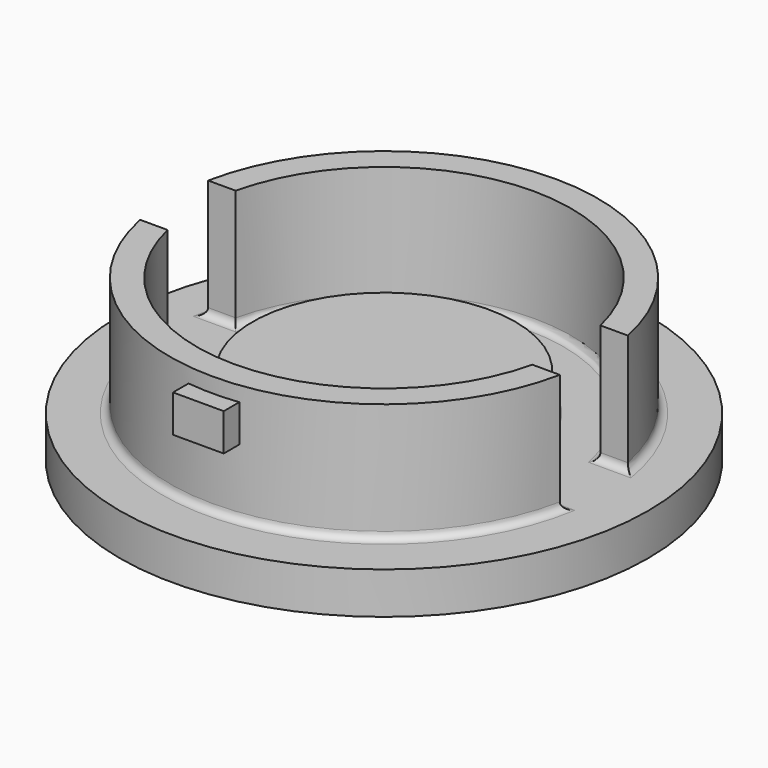
from build123d import *

# Parameters (mm, degrees)
F0_R         = 8.85
F1_DEPTH     = 1.4
F2_R         = 7.175
F2_R_2       = 6.275
F3_DEPTH     = 4
F5_W         = 2.85
F5_H         = 4
F6_DEPTH     = 25
F7_R         = 4.4
F8_DEPTH     = 1.27
F10_W        = 1.7
F10_H        = 1.25
F11_DEPTH    = 0.6
F12_W        = 12.45
F12_H        = 1.85
F13_DEPTH    = 0.8
F14_T1_DEPTH = 6.7489794856
F15_R        = 0.25


# Not quite as in the source:
# - a fillet or chamfer that OpenCascade refuses, or shapes differently, is made with other operations: its cross-section is extruded or revolved along the edge and cut away or added
# - a pattern or mirror of a feature is missing from the dataset's text; its kind, count and spacing are read off the source's solid


with BuildPart() as f1:
    # F0 (on Top) → F1 (new body)
    with BuildSketch(Plane.XY):
        Circle(F0_R)
    extrude(amount=F1_DEPTH)

    # F2 (on face) → F3 (join)
    with BuildSketch(Plane.XY.offset(1.4)):
        Circle(F2_R)
        Circle(F2_R_2, mode=Mode.SUBTRACT)
    extrude(amount=F3_DEPTH)

    # F5 (on offset) → F6 (cut)
    with BuildSketch(Plane.YZ.offset(7.175)):
        with Locations((0, 3.4)):
            Rectangle(F5_W, F5_H)
    extrude(amount=-F6_DEPTH, mode=Mode.SUBTRACT)

    # F7 (on face) → F8 (join)
    with BuildSketch(Plane.XY.offset(1.4)):
        Circle(F7_R)
    extrude(amount=F8_DEPTH)

    # F10 (on offset) → F11 (join, symmetric)
    with BuildSketch(Plane.XZ.offset(7.175)):
        with Locations((0, 4.275)):
            Rectangle(F10_W, F10_H)
    f11 = extrude(amount=F11_DEPTH, both=True)

    # F11_copies: F11 across plane
    add(f11.mirror(Plane.ZX))

    # F12 (on face) → F13 (cut)
    with BuildSketch(Plane(origin=(0, 0, 0), x_dir=(1, 0, 0), z_dir=(0, 0, -1))):
        Rectangle(F12_W, F12_H)
    extrude(amount=-F13_DEPTH, mode=Mode.SUBTRACT)

    # F14: fillet of radius 1 on 2 edges, made by hand

    # F14_s2 → F14_t1 (join)
    with BuildSketch(Plane.XZ.offset(-3.3744897428)):
        with BuildLine():
            ThreePointArc((-6.225, 0), (-5.8776596349, 0.5745966692), (-5.2452041029, 0.8))
            Line((-5.2452041029, 0.8), (-6.225, 0.8))
            Line((-6.225, 0.8), (-6.225, 0))
        make_face()
        with BuildLine():
            ThreePointArc((6.225, 0), (5.8776596349, 0.5745966692), (5.2452041029, 0.8))
            Line((5.2452041029, 0.8), (6.225, 0.8))
            Line((6.225, 0.8), (6.225, 0))
        make_face()
    extrude(amount=F14_T1_DEPTH)

    # F15
    f15_edges = [f1.edges().sort_by_distance(p)[0] for p in [
        (0, 6.275, 1.4),
        (6.571562, 1.425, 1.4),
        (-6.571562, 1.425, 1.4),
        (0, 7.175, 1.4),
        (-4.4, 0, 1.4),
        (-6.571562, -1.425, 1.4),
        (6.571562, -1.425, 1.4),
        (0, -7.175, 1.4),
        (0, -6.275, 1.4),
    ]]
    fillet(f15_edges, radius=F15_R)


solid = f1.part
